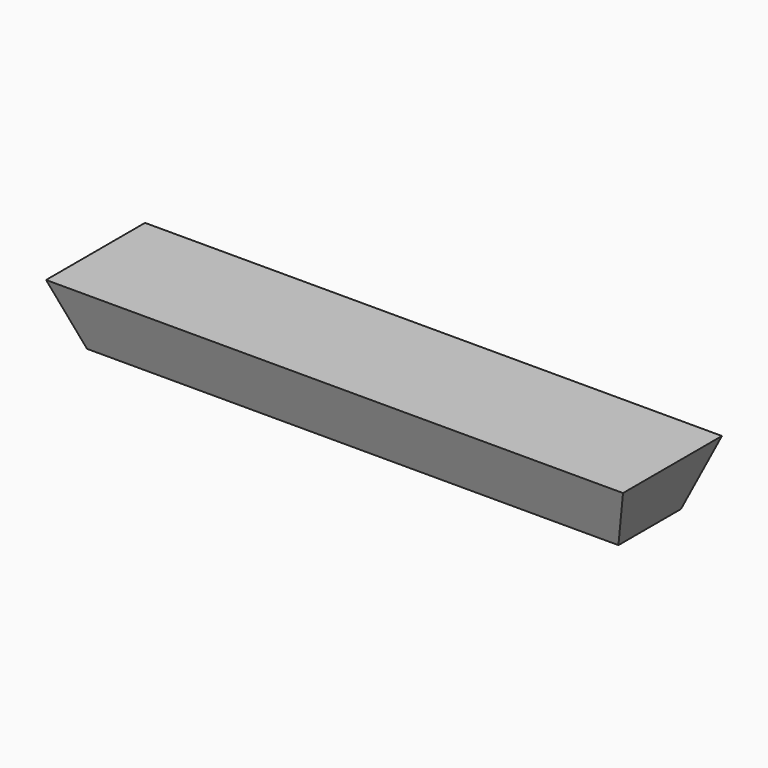
from build123d import *

# Parameters (mm, degrees)
F1_W     = 340
F1_H     = 50
F2_DEPTH = 40
F2_TAPER = -20


with BuildPart() as f2:
    # F1 (on face) → F2 (new body)
    with BuildSketch(Plane.XY):
        with Locations((4.195868969, -44.5757127798)):
            Rectangle(F1_W, F1_H)
    extrude(amount=F2_DEPTH, taper=F2_TAPER)


solid = f2.part
